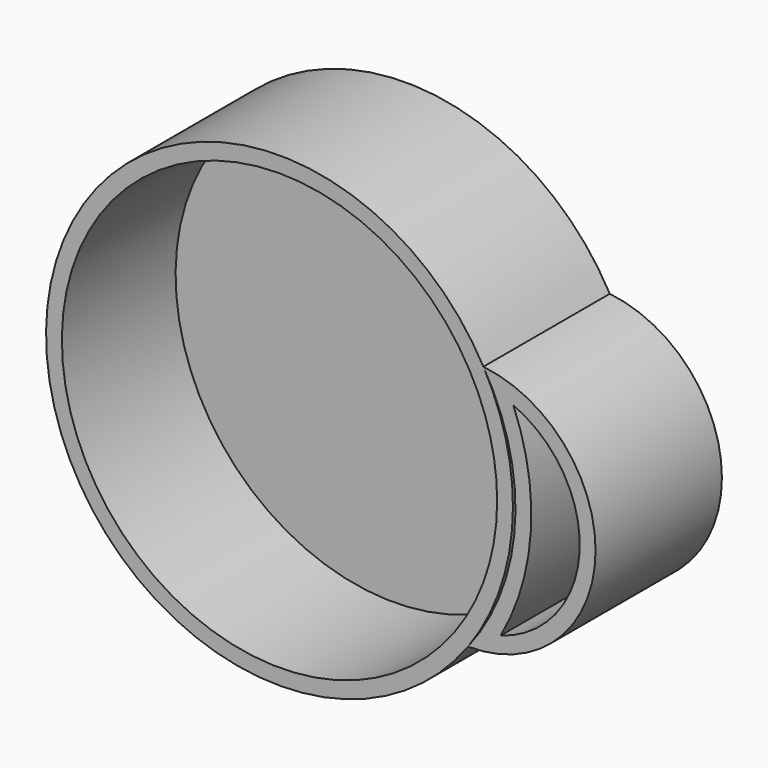
from build123d import *

# Parameters (mm, degrees)
F1_DEPTH = 25.4
F2_T     = -2.54
F2_2_T   = -2.54


with BuildPart() as f1:
    # F0 (on Front) → F1 (new body)
    with BuildSketch(Plane.XZ):
        with BuildLine():
            ThreePointArc((7.4890239755, 3.3776608035), (12.8672812185, 13.8780094101), (14.7210613775, 25.529038161))
            ThreePointArc((14.7210613775, 25.529038161), (13.5144494489, 34.9702915027), (9.9721789394, 43.8046277339))
            ThreePointArc((9.9721789394, 43.8046277339), (-60.2889464795, 27.8305479659), (7.4890239755, 3.3776608035))
        make_face()
    extrude(amount=F1_DEPTH)

    # F2#2
    f2_2_openings = [f1.faces().sort_by_distance(p)[0] for p in [
        (-22.819251, -25.4, 25.529038),
    ]]
    offset(amount=F2_2_T, openings=f2_2_openings)


with BuildPart() as f1b:
    # F0 (on Front) → F1, piece 2 (new body)
    with BuildSketch(Plane.XZ):
        with BuildLine():
            ThreePointArc((7.4890239755, 3.3776608035), (27.9674398386, 22.4095554842), (9.9721789394, 43.8046277339))
            ThreePointArc((9.9721789394, 43.8046277339), (15.0657511021, 23.2020189031), (7.4890239755, 3.3776608035))
        make_face()
    extrude(amount=F1_DEPTH)

    # F2
    f2_openings = [f1b.faces().sort_by_distance(p)[0] for p in [
        (19.125855, -25.4, 22.952634),
    ]]
    offset(amount=F2_T, openings=f2_openings)


solid = Compound([f1.part, f1b.part])
